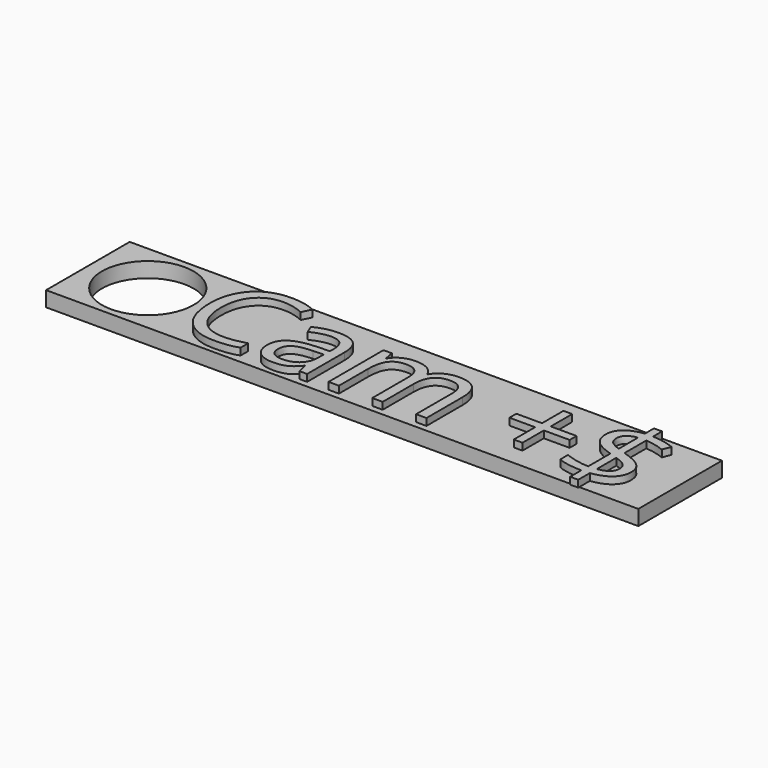
from build123d import *

# Parameters (mm, degrees)
F0_W         = 86.36
F0_H         = 15.24
F0_R         = 6.6763850661
F1_DEPTH     = 2.2098
F2_TEXT_SIZE = 18.7088677194
F3_DEPTH     = 1.016


# Not quite as in the source:
# - Text() gives the source's letters only with a copy of the font that has no kerning and outlines rounded to 1/6400 em; it was checked with that copy


with BuildPart() as f1:
    # F0 (on Top) → F1 (new body)
    with BuildSketch(Plane.XY):
        Rectangle(F0_W, F0_H)
        with Locations((-34.4500094652, 0)):
            Circle(F0_R, mode=Mode.SUBTRACT)
    extrude(amount=F1_DEPTH)

    # F2 (on face) → F3 (join)
    with BuildSketch(Plane.XY.offset(2.2098)):
        with Locations((-26.5309214592, -6.7154457793)):
            Text('Cam +$', F2_TEXT_SIZE, font='Open Sans', text_align=(TextAlign.LEFT, TextAlign.BOTTOM))
    extrude(amount=F3_DEPTH)


solid = f1.part
